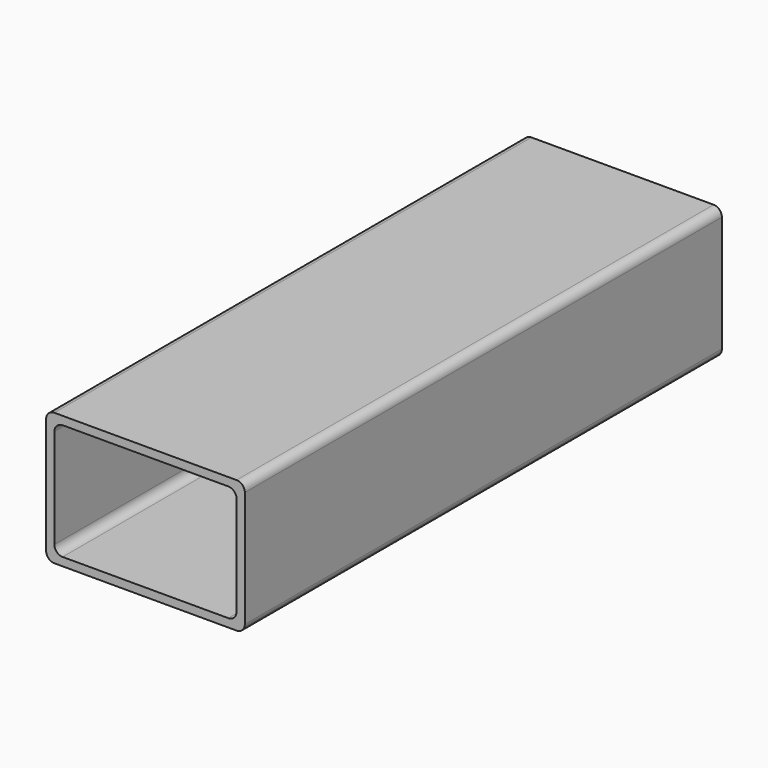
from build123d import *

# Parameters (mm, degrees)
F0_W     = 76.2
F0_H     = 50.8
F0_W_2   = 69.85
F0_H_2   = 44.45
F2_DEPTH = 228.6
F3_R     = 3.175


# Not quite as in the source:
# - a variable given as a bare number and used for a length is read in inches; the dataset says mm whatever the document's units were


with BuildPart() as f2:
    # F0 (on Front) → F2 (new body)
    with BuildSketch(Plane.XZ):
        Rectangle(F0_W, F0_H)
        Rectangle(F0_W_2, F0_H_2, mode=Mode.SUBTRACT)
    extrude(amount=F2_DEPTH)

    # F3
    f3_edges = [f2.edges().sort_by_distance(p)[0] for p in [
        (-38.1, -114.3, 25.4),
        (38.1, -114.3, 25.4),
        (38.1, -114.3, -25.4),
        (-38.1, -114.3, -25.4),
        (-34.925, -114.3, -22.225),
        (-34.925, -114.3, 22.225),
        (34.925, -114.3, 22.225),
        (34.925, -114.3, -22.225),
    ]]
    fillet(f3_edges, radius=F3_R)


solid = f2.part
